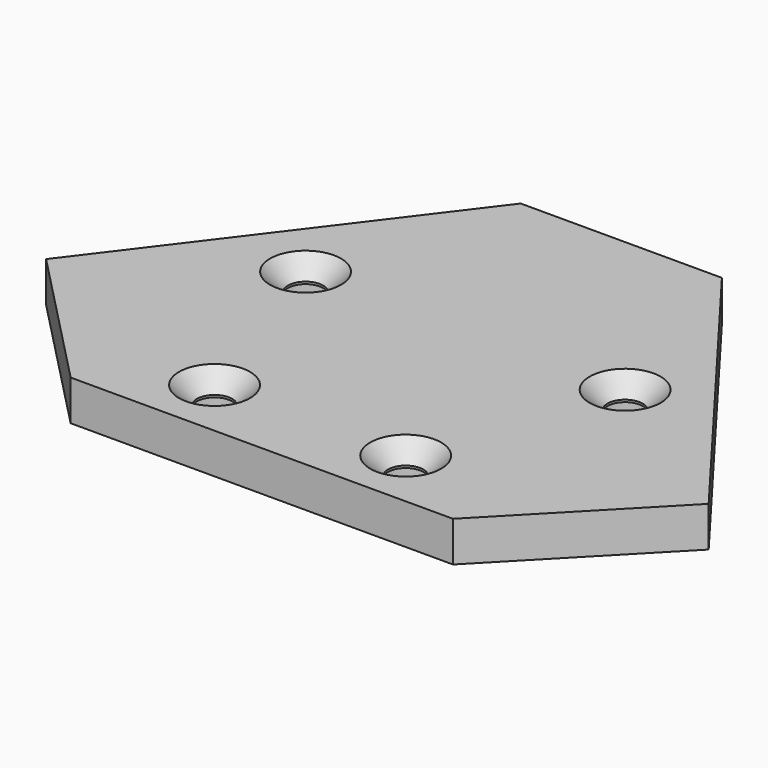
from build123d import *

# Parameters (mm, degrees)
F0_R     = 3.5
F1_DEPTH = 4
F0_R_2   = 1.75
F2_DEPTH = 4
F3_SIZE  = 1.78
F4_DEPTH = 2


# Not quite as in the source:
# - a feature names something its author has since deleted; it is built from what else it names


with BuildPart() as f1:
    # F0 (on Top) → F1 (new body)
    with BuildSketch(Plane.XY):
        Polygon((0, 44.6608208763), (0, 0), (19, 0), (32.9255871796, 14.3554178519), (10, 44.6608208763), align=None)
        with Locations((9.5, 6)):
            Circle(F0_R, mode=Mode.SUBTRACT)
        with Locations((15.8802193485, 25.2849848836)):
            Circle(F0_R, mode=Mode.SUBTRACT)
        Polygon((-9.5, 0), (0, 0), (0, 44.6608208763), (-10, 44.6608208763), (-32.9255871796, 14.3554178519), (-19, 0), align=None)
        with Locations((-9.5, 6)):
            Circle(F0_R, mode=Mode.SUBTRACT)
        with Locations((-15.8802193485, 25.2849848836)):
            Circle(F0_R, mode=Mode.SUBTRACT)
    extrude(amount=F1_DEPTH)

    # F0 (on Top) → F2 (join)
    with BuildSketch(Plane.XY):
        with Locations((9.5, 6)):
            Circle(F0_R)
        with Locations((9.5, 6)):
            Circle(F0_R_2, mode=Mode.SUBTRACT)
        with Locations((-9.5, 6)):
            Circle(F0_R)
        with Locations((-9.5, 6)):
            Circle(F0_R_2, mode=Mode.SUBTRACT)
        with Locations((-15.8802193485, 25.2849848836)):
            Circle(F0_R)
        with Locations((-15.8802193485, 25.2849848836)):
            Circle(F0_R_2, mode=Mode.SUBTRACT)
        with Locations((15.8802193485, 25.2849848836)):
            Circle(F0_R)
        with Locations((15.8802193485, 25.2849848836)):
            Circle(F0_R_2, mode=Mode.SUBTRACT)
    extrude(amount=F2_DEPTH)

    # F3
    f3_edges = [f1.edges().sort_by_distance(p)[0] for p in [
        (14.130219, 25.284985, 4),
        (-17.630219, 25.284985, 4),
        (-11.25, 6, 4),
        (7.75, 6, 4),
    ]]
    chamfer(f3_edges, length=F3_SIZE)

    # F0 (on Top) → F4 (cut)
    with BuildSketch(Plane.XY):
        with Locations((-15.8802193485, 25.2849848836)):
            Circle(F0_R)
        with Locations((-15.8802193485, 25.2849848836)):
            Circle(F0_R_2, mode=Mode.SUBTRACT)
        with Locations((15.8802193485, 25.2849848836)):
            Circle(F0_R)
        with Locations((15.8802193485, 25.2849848836)):
            Circle(F0_R_2, mode=Mode.SUBTRACT)
        with Locations((9.5, 6)):
            Circle(F0_R)
        with Locations((9.5, 6)):
            Circle(F0_R_2, mode=Mode.SUBTRACT)
        with Locations((-9.5, 6)):
            Circle(F0_R)
        with Locations((-9.5, 6)):
            Circle(F0_R_2, mode=Mode.SUBTRACT)
    extrude(amount=F4_DEPTH, mode=Mode.SUBTRACT)


solid = f1.part
